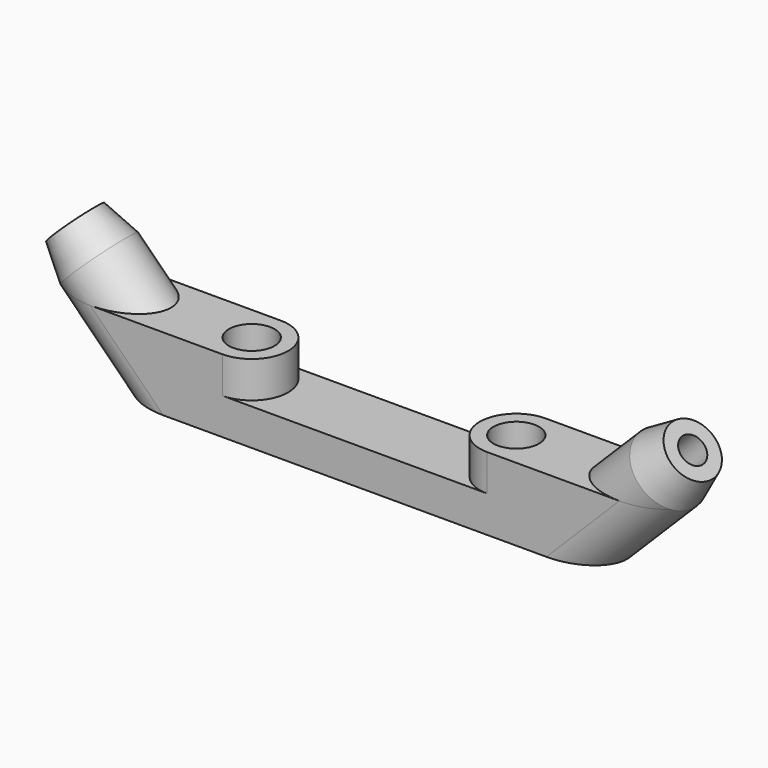
from build123d import *

# Parameters (mm, degrees)
F1_DEPTH  = 4
F2_R      = 3.99999
F3_R      = 2.5
F4_DEPTH  = 8
F6_DEPTH  = 4
F9_R      = 4
F10_DEPTH = 6.851053331


# Not quite as in the source:
# - a fillet or chamfer that OpenCascade refuses, or shapes differently, is made with other operations: its cross-section is extruded or revolved along the edge and cut away or added
# - a fillet or chamfer is up to 0.001 mm smaller than in the source, because OpenCascade refuses the exact size


with BuildPart() as f1:
    # F0 (on Front) → F1 (new body, symmetric)
    with BuildSketch(Plane.XZ):
        Polygon((-26.6568542495, 0), (0, 0), (0, 8), (-34.6568542495, 8), align=None)
    extrude(amount=F1_DEPTH, both=True)

    # F2 (radius 4 in the source; OpenCascade refuses exactly that, so slightly less here)
    f2_edges = [f1.edges().sort_by_distance(p)[0] for p in [
        (-30.656854, 4, 4),
        (-30.656854, -4, 4),
    ]]
    fillet(f2_edges, radius=F2_R)

    # F3 (on face) → F4 (cut, through all)
    with BuildSketch(Plane.XY.offset(8)):
        with Locations((-14.5, 0)):
            Circle(F3_R)
    extrude(amount=-F4_DEPTH, mode=Mode.SUBTRACT)

    # F5 (on face) → F6 (cut)
    with BuildSketch(Plane.XY.offset(8)):
        with BuildLine():
            ThreePointArc((-14.5, 4), (-10.5, 0), (-14.5, -4))
            Line((-14.5, -4), (0, -4))
            Line((0, -4), (0, 4))
            Line((0, 4), (-14.5, 4))
        make_face()
    extrude(amount=-F6_DEPTH, mode=Mode.SUBTRACT)

    # F9 (on line) → F10 (join, symmetric)
    with BuildSketch(Plane(origin=(-18.5, 0, 18.5), x_dir=(0, 1, 0), z_dir=(0.7071067812, 0, -0.7071067812))):
        with Locations((0, -14.8492424049)):
            Circle(F9_R)
    extrude(amount=F10_DEPTH, both=True)

    # F7 (on Front) → F11 (revolve, cut)
    with BuildSketch(Plane.XZ):
        Polygon((-20.5108239612, -2.6104963823), (-19.4501637894, -1.5498362106), (-43.5361095251, 22.5361095251), (-44.5967696969, 21.4754493533), align=None)
    revolve(axis=Axis((-31.4931366573, 0, 10.4931366573), (-0.7071067812, 0, 0.7071067812)), mode=Mode.SUBTRACT)

    # F12: chamfer of 1 x 3.7320508076 on 1 edges, made by hand

    # F12_s1 → F12_t2 (revolve, cut)
    with BuildSketch(Plane(origin=(-10.5, 0, -10.5), x_dir=(0, 1, 0), z_dir=(-0.7071067812, 0, -0.7071067812))):
        Polygon((4, -29.2819534274), (3, -33.0140042349), (4, -33.0140042349), align=None)
    revolve(axis=Axis((-33.8444262687, 0, 12.8444262687), (0.7071067812, 0, -0.7071067812)), mode=Mode.SUBTRACT)

    # F13: F1 across face


with BuildPart() as f1_1:
    add(f1.part)
    add(f1.part.mirror(Plane(origin=(0, 0, 2), x_dir=(0, 1, 0), z_dir=(1, 0, 0))))


solid = f1_1.part
